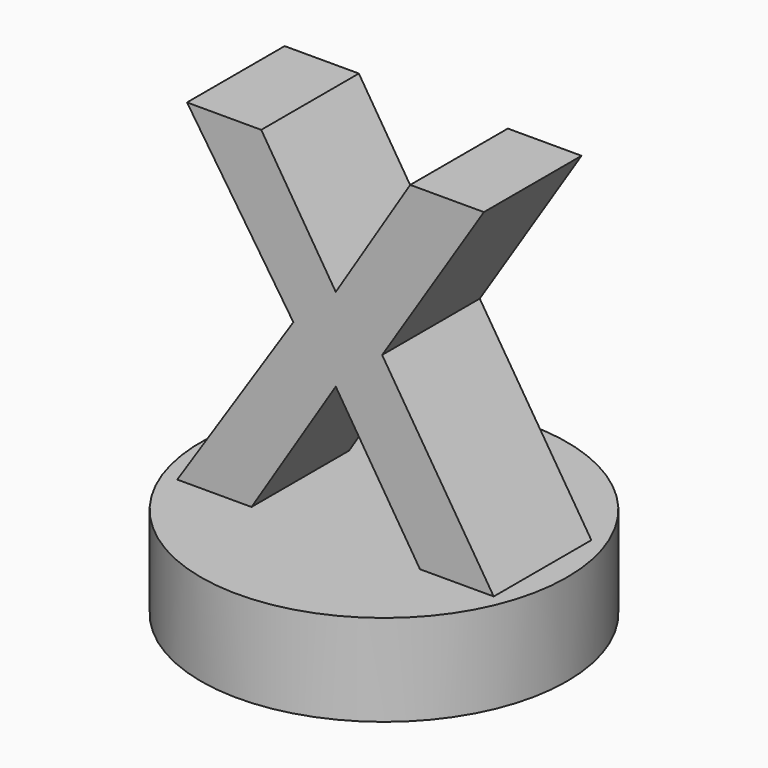
from build123d import *

# Parameters (mm, degrees)
F0_R          = 6
F1_DEPTH      = 3
F2_TEXT_SIZE  = 15.9722222222
F3_DEPTH      = 2
F3_DEPTH_BACK = 2


# Not quite as in the source:
# - Text() gives the source's letters only with a copy of the font that has no kerning and outlines rounded to 1/6400 em; it was checked with that copy


with BuildPart() as f1:
    # F0 (on Top) → F1 (new body)
    with BuildSketch(Plane.XY):
        Circle(F0_R)
    extrude(amount=-F1_DEPTH)

    # F2 (on Front) → F3 (join, two sides)
    with BuildSketch(Plane.XZ) as f3_sk:
        with Locations((-5.3166919338, 0)):
            Text('X', F2_TEXT_SIZE, font='Arimo', font_style=FontStyle.BOLD, text_align=(TextAlign.LEFT, TextAlign.BOTTOM))
    extrude(amount=F3_DEPTH)
    extrude(f3_sk.sketch, amount=-F3_DEPTH_BACK)


solid = f1.part
